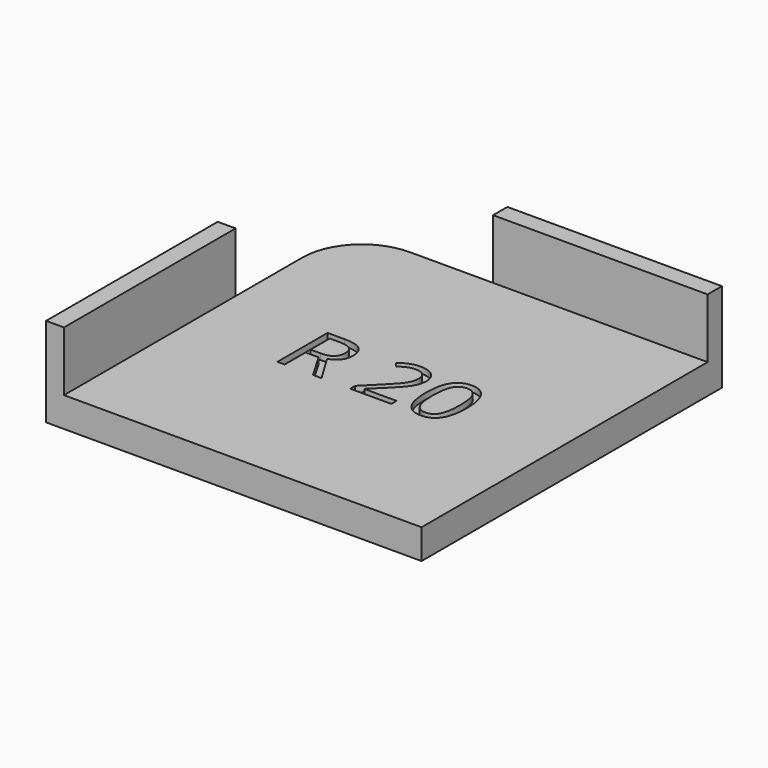
from build123d import *

# Parameters (mm, degrees)
F1_DEPTH      = 5
F2_W          = 3
F2_H          = 36
F2_W_2        = 36
F2_H_2        = 3
F3_DEPTH      = 10
F3_DEPTH_BACK = 5
F4_TEXT_SIZE  = 14.7307043118
F5_DEPTH      = 1


# Not quite as in the source:
# - Text() gives the source's letters only with a copy of the font that has no kerning and outlines rounded to 1/6400 em; it was checked with that copy


with BuildPart() as f1:
    # F0 (on Top) → F1 (new body)
    with BuildSketch(Plane.XY):
        with BuildLine():
            Line((50, 10), (0, 10))
            ThreePointArc((0, 10), (-7.0710678119, 7.0710678119), (-10, 0))
            Line((-10, 0), (-10, -50))
            Line((-10, -50), (50, -50))
            Line((50, -50), (50, 10))
        make_face()
    extrude(amount=F1_DEPTH)

    # F2 (on face) → F3 (join, two sides)
    with BuildSketch(Plane.XY.offset(5)) as f3_sk:
        with Locations((-11.5, -32)):
            Rectangle(F2_W, F2_H)
        with Locations((32, 11.5)):
            Rectangle(F2_W_2, F2_H_2)
    extrude(amount=F3_DEPTH)
    extrude(f3_sk.sketch, amount=-F3_DEPTH_BACK)

    # F4 (on face) → F5 (cut)
    with BuildSketch(Plane.XY.offset(5)):
        with Locations((4.4858261352, -25.144356166)):
            Text('R 20', F4_TEXT_SIZE, font='Open Sans', text_align=(TextAlign.LEFT, TextAlign.BOTTOM))
    extrude(amount=-F5_DEPTH, mode=Mode.SUBTRACT)


with BuildPart() as f6_1:
    # F6: copy of F1
    add(f1.part)


solid = f6_1.part
